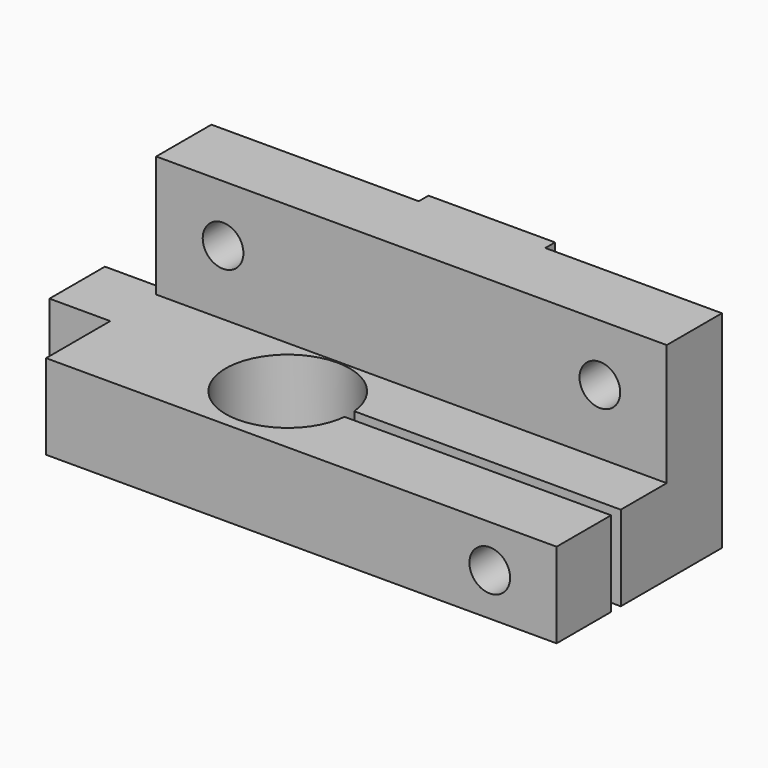
from build123d import *

# Parameters (mm, degrees)
F0_W          = 42
F0_H          = 17
F1_DEPTH      = 7
F4_DEPTH      = 25
F5_W          = 42
F5_H          = 5.6745335534
F6_DEPTH      = 10
F7_R          = 1.675
F8_DEPTH      = 25
F9_DEPTH      = 25
F10_TEXT_SIZE = 23.6111111111
F11_DEPTH     = 1
F12_W         = 5.7
F12_H         = 7
F13_DEPTH     = 5


# Not quite as in the source:
# - Text() gives the source's letters only with a copy of the font that has no kerning and outlines rounded to 1/6400 em; it was checked with that copy


with BuildPart() as f1:
    # F0 (on Top) → F1 (new body)
    with BuildSketch(Plane.XY):
        with Locations((21, 8.5)):
            Rectangle(F0_W, F0_H)
    extrude(amount=F1_DEPTH)

    # F3 (on face) → F4 (cut)
    with BuildSketch(Plane(origin=(0, 17, 0), x_dir=(-1, 0, 0), z_dir=(0, 1, 0))):
        with BuildLine():
            ThreePointArc((-38.175, 3.5), (-36.5, 1.825), (-34.825, 3.5))
            ThreePointArc((-34.825, 3.5), (-36.5, 5.175), (-38.175, 3.5))
        make_face()
    extrude(amount=-F4_DEPTH, mode=Mode.SUBTRACT)

    # F5 (on face) → F6 (join)
    with BuildSketch(Plane.XY.offset(7)):
        with Locations((21, 14.1627332233)):
            Rectangle(F5_W, F5_H)
    extrude(amount=F6_DEPTH)

    # F7 (on face) → F8 (cut)
    with BuildSketch(Plane(origin=(0, 17, 0), x_dir=(-1, 0, 0), z_dir=(0, 1, 0))):
        with Locations((-36.5, 12.325)):
            Circle(F7_R)
        with Locations((-5.5, 12.325)):
            Circle(F7_R)
    extrude(amount=-F8_DEPTH, mode=Mode.SUBTRACT)

    # F2 (on face) → F9 (cut)
    with BuildSketch(Plane.XY.offset(7)):
        with BuildLine():
            ThreePointArc((20.0754310162, 5.6), (20.0938540508, 5.8496983645), (20.1, 6.1))
            ThreePointArc((20.1, 6.1), (20.0938540508, 6.3503016355), (20.0754310162, 6.6))
            ThreePointArc((20.0754310162, 6.6), (9.9, 6.1), (20.0754310162, 5.6))
        make_face()
        with BuildLine():
            Line((42, 6.1), (20.1, 6.1))
            ThreePointArc((20.1, 6.1), (20.0938540508, 5.8496983645), (20.0754310162, 5.6))
            Line((20.0754310162, 5.6), (42, 5.6))
            Line((42, 5.6), (42, 6.1))
        make_face()
        with BuildLine():
            ThreePointArc((20.0754310162, 6.6), (20.0938540508, 6.3503016355), (20.1, 6.1))
            Line((20.1, 6.1), (42, 6.1))
            Line((42, 6.1), (42, 6.6))
            Line((42, 6.6), (20.0754310162, 6.6))
        make_face()
    extrude(amount=-F9_DEPTH, mode=Mode.SUBTRACT)

    # F10 (on face) → F11 (join)
    with BuildSketch(Plane(origin=(0, 17, 0), x_dir=(-1, 0, 0), z_dir=(0, 1, 0))):
        with Locations(Location((-14.9393391335, 17), (0, 0, -180))):
            Text('L', F10_TEXT_SIZE, font='Open Sans', font_style=FontStyle.BOLD, text_align=(TextAlign.LEFT, TextAlign.BOTTOM))
    extrude(amount=F11_DEPTH)

    # F12 (on face) → F13 (join)
    with BuildSketch(Plane(origin=(0, 0, 0), x_dir=(0, -1, 0), z_dir=(-1, 0, 0))):
        with Locations((-9.45, 3.5)):
            Rectangle(F12_W, F12_H)
    extrude(amount=F13_DEPTH)


solid = f1.part
